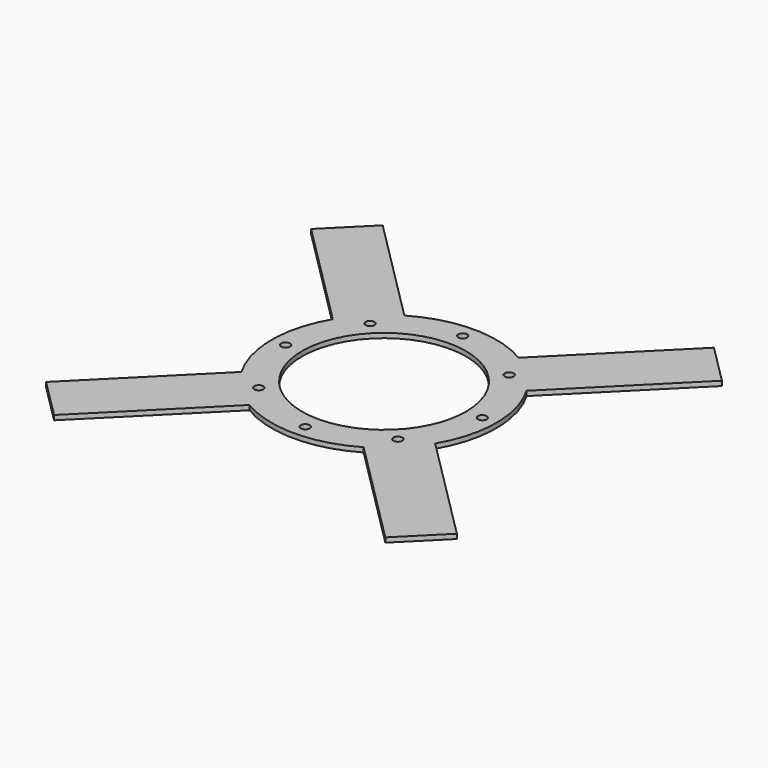
from build123d import *

# Parameters (mm, degrees)
F1_DEPTH        = 6.35
F2_R            = 6.0325
F3_DEPTH        = 25.4
F3_COPIES_COUNT = 8


# Not quite as in the source:
# - a pattern or mirror of a feature is missing from the dataset's text; its kind, count and spacing are read off the source's solid


with BuildPart() as f1:
    # F0 (on Top) → F1 (new body)
    with BuildSketch(Plane.XY):
        with BuildLine():
            Line((-278.3879397531, 224.5064030267), (-131.2819155679, 77.4003788415))
            ThreePointArc((-131.2819155679, 77.4003788415), (-152.4, 0), (-131.2819155679, -77.4003788415))
            Line((-131.2819155679, -77.4003788415), (-278.3879397531, -224.5064030267))
            Line((-278.3879397531, -224.5064030267), (-224.5064030267, -278.3879397531))
            Line((-224.5064030267, -278.3879397531), (-77.4003788415, -131.2819155679))
            ThreePointArc((-77.4003788415, -131.2819155679), (0, -152.4), (77.4003788415, -131.2819155679))
            Line((77.4003788415, -131.2819155679), (224.5064030267, -278.3879397531))
            Line((224.5064030267, -278.3879397531), (278.3879397531, -224.5064030267))
            Line((278.3879397531, -224.5064030267), (131.2819155679, -77.4003788415))
            ThreePointArc((131.2819155679, -77.4003788415), (152.4, 0), (131.2819155679, 77.4003788415))
            Line((131.2819155679, 77.4003788415), (278.3879397531, 224.5064030267))
            Line((278.3879397531, 224.5064030267), (224.5064030267, 278.3879397531))
            Line((224.5064030267, 278.3879397531), (77.4003788415, 131.2819155679))
            ThreePointArc((77.4003788415, 131.2819155679), (0, 152.4), (-77.4003788415, 131.2819155679))
            Line((-77.4003788415, 131.2819155679), (-224.5064030267, 278.3879397531))
            Line((-224.5064030267, 278.3879397531), (-278.3879397531, 224.5064030267))
        make_face()
        with BuildLine():
            ThreePointArc((100.7552507667, -46.8737140403), (-108.5015964547, 24.0035245698), (111.125, 0))
            ThreePointArc((111.125, 0), (108.5015964547, -24.0035245698), (100.7552507667, -46.8737140403))
        make_face(mode=Mode.SUBTRACT)
    extrude(amount=F1_DEPTH)

    # F2 (on face) → F3 (cut)
    with BuildSketch(Plane.XY.offset(6.35)):
        with Locations((-133.35, 0)):
            Circle(F2_R)
    f3 = extrude(amount=-F3_DEPTH, mode=Mode.SUBTRACT)

    # F3_copies: F3 ×8 about axis
    f3_copies_axis = Axis((0, 0, 0), (0, 0, 1))
    for i in range(1, F3_COPIES_COUNT):
        add(f3.rotate(f3_copies_axis, i * 360 / F3_COPIES_COUNT), mode=Mode.SUBTRACT)


solid = f1.part
